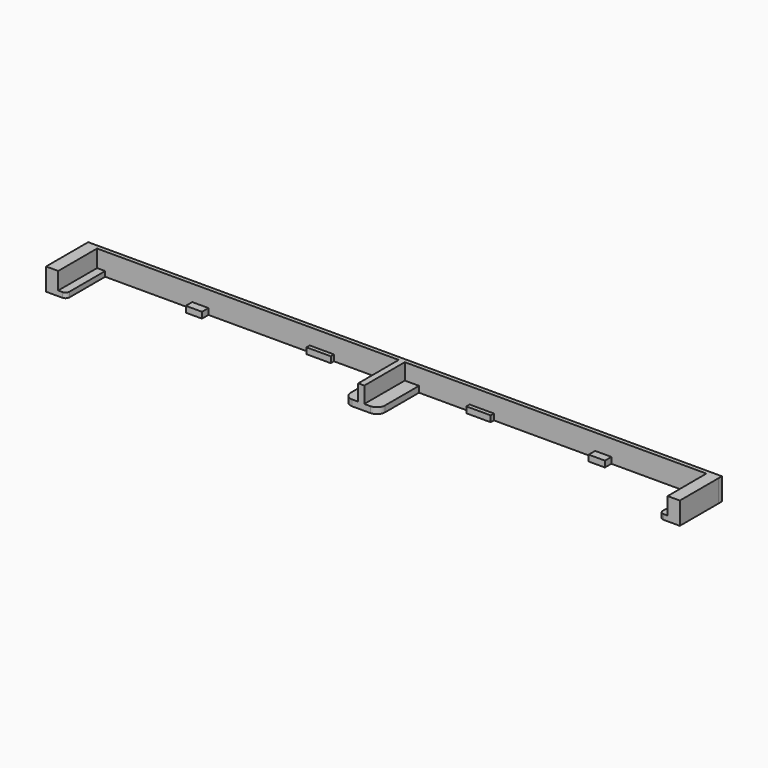
from build123d import *

# Parameters (mm, degrees)
F0_W     = 2.4
F0_H     = 9.6
F0_H_2   = 0.8
F0_W_2   = 1.2
F0_H_3   = 10
F0_W_3   = 1.6
F1_DEPTH = 4.4
F0_W_4   = 3.2
F0_H_4   = 1.6
F0_W_5   = 4.8
F2_DEPTH = 1.2
F3_DEPTH = 1


# Not quite as in the source:
# - ends of sketch curves that miss each other by under 0.0002 mm in the source are joined


with BuildPart() as f1:
    # F0 (on Top) → F1 (new body)
    with BuildSketch(Plane.XY):
        with Locations((-61.4, 0.5979961667)):
            Rectangle(F0_W, F0_H)
        with Locations((-61.4, 5.7979961667)):
            Rectangle(F0_W, F0_H_2)
        Polygon((-58.6, 5.3979961667), (-41.4000016928, 5.3979961667), (-38.2000016928, 5.3979961667), (-18.2000016928, 5.3979961667), (-13.4000016928, 5.3979961667), (-3.4000016928, 5.3979961667), (-0.6092149836, 5.3979961667), (0.5907850164, 5.3979961667), (3.3999983072, 5.3979961667), (13.4000016928, 5.3979961667), (18.2000016928, 5.3979961667), (38.2000016928, 5.3979961667), (41.4000016928, 5.3979961667), (58.6059018172, 5.3979961667), (58.6063936353, 6.1979961667), (-58.6, 6.1979961667), align=None)
        Polygon((62.5999775911, 6.1979961667), (60.1678602397, 6.1979961667), (60.1701559369, 5.3979961667), (62.5999775911, 5.3979961667), (62.5999775911, 5.7979961667), align=None)
        Polygon((62.5999775911, 5.3979961667), (60.1701559369, 5.3979961667), (60.1977043028, -4.2020038333), (62.6, -4.2020038333), align=None)
        with Locations((-0.0092149836, 0.3979961667)):
            Rectangle(F0_W_2, F0_H_3)
        with Locations((-59.4, 5.7979961667)):
            Rectangle(F0_W_3, F0_H_2)
        Polygon((60.1678602397, 6.1979961667), (58.6063936353, 6.1979961667), (58.6059018172, 5.3979961667), (60.1701559369, 5.3979961667), align=None)
    extrude(amount=F1_DEPTH)

    # F0 (on Top) → F2 (join)
    with BuildSketch(Plane.XY):
        with Locations((39.8000016928, 4.5979961667)):
            Rectangle(F0_W_4, F0_H_4)
        with Locations((15.8000016928, 4.9979961667)):
            Rectangle(F0_W_5, F0_H_2)
        with BuildLine():
            Line((3.3999983072, 5.3979961667), (0.5907850164, 5.3979961667))
            Line((0.5907850164, 5.3979961667), (0.5907850164, -4.6020038333))
            Line((0.5907850164, -4.6020038333), (1.7999983072, -4.6020038333))
            ThreePointArc((1.7999983072, -4.6020038333), (2.9313691571, -4.1333746832), (3.3999983072, -3.0020038333))
            Line((3.3999983072, -3.0020038333), (3.3999983072, 5.3979961667))
        make_face()
        with BuildLine():
            Line((-0.6092149836, 5.3979961667), (-3.4000016928, 5.3979961667))
            Line((-3.4000016928, 5.3979961667), (-3.4000016928, -3.0020038333))
            ThreePointArc((-3.4000016928, -3.0020038333), (-2.9313725427, -4.1333746832), (-1.8000016928, -4.6020038333))
            Line((-1.8000016928, -4.6020038333), (-0.6092149836, -4.6020038333))
            Line((-0.6092149836, -4.6020038333), (-0.6092149836, 5.3979961667))
        make_face()
        with Locations((-15.8000016928, 4.9979961667)):
            Rectangle(F0_W_5, F0_H_2)
        with Locations((-39.8000016928, 4.5979961667)):
            Rectangle(F0_W_4, F0_H_4)
    extrude(amount=F2_DEPTH)

    # F0 (on Top) → F3 (join)
    with BuildSketch(Plane.XY):
        with BuildLine():
            Line((-58.6, -3.4020038333), (-58.6, 5.3979961667))
            Line((-58.6, 5.3979961667), (-60.2, 5.3979961667))
            Line((-60.2, 5.3979961667), (-60.2, -4.2020038333))
            Line((-60.2, -4.2020038333), (-59.4, -4.2020038333))
            ThreePointArc((-59.4, -4.2020038333), (-58.8343145751, -3.9676892582), (-58.6, -3.4020038333))
        make_face()
        with BuildLine():
            Line((60.1701559369, 5.3979961667), (58.6059018172, 5.3979961667))
            Line((58.6059018172, 5.3979961667), (58.6004748691, -3.4295733769))
            ThreePointArc((58.6004748691, -3.4295733769), (58.8441470155, -3.9773540027), (59.3999996781, -4.2020038333))
            Line((59.3999996781, -4.2020038333), (60.1977043028, -4.2020038333))
            Line((60.1977043028, -4.2020038333), (60.1701559369, 5.3979961667))
        make_face()
    extrude(amount=F3_DEPTH)


solid = f1.part
